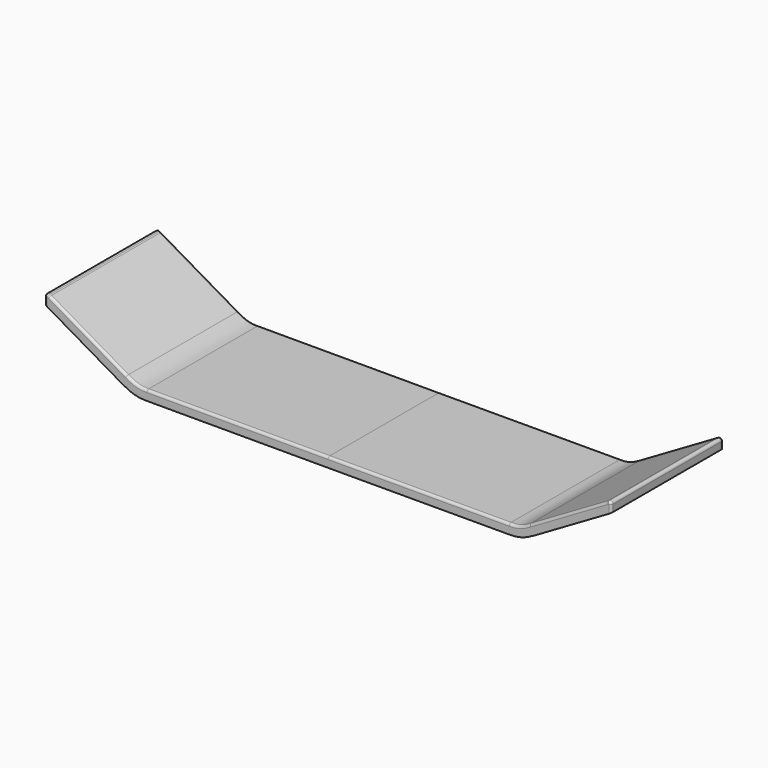
from build123d import *

# Parameters (mm, degrees)
F1_DEPTH = 146.05
F2_R     = 2.54


with BuildPart() as f1:
    # F0 (on Front) → F1 (new body)
    with BuildSketch(Plane.XZ):
        with BuildLine():
            Line((1.5943159571, 65.9026825806), (1.5943159571, 54.15516499))
            Line((1.5943159571, 54.15516499), (81.9025710225, 7.5405244716))
            add(Edge.make_bspline(
                [(81.9025710225, 7.5405244716), (92.2999233007, 1.5054497635), (98.6241698265, 0), (108.1725358963, 0)],
                knots=[0, 0, 0, 0, 27.3307622246, 27.3307622246, 27.3307622246, 27.3307622246], degree=3))
            Line((108.1725358963, 0), (138.4361670146, -1.768e-06))
            Line((138.4361670146, -1.768e-06), (163.8361670146, -3.2519e-06))
            Line((163.8361670146, -3.2519e-06), (297.1861670146, -1.10422e-05))
            Line((297.1861670146, -1.10422e-05), (297.1800001915, 10.1599889582))
            Line((297.1800001915, 10.1599889582), (108.1725311829, 10.16))
            add(Edge.make_bspline(
                [(87.0029644932, 16.3275368446), (88.188553852, 15.6393696939), (90.394248444, 14.4210715589), (93.2713691382, 13.0231304302), (95.7978416249, 11.994384017), (98.0869107324, 11.2602812726), (100.2922847586, 10.7469020057), (102.5915460742, 10.4019914085), (105.1499671195, 10.2020688941), (107.1124775165, 10.1600000624), (108.1725311829, 10.16)],
                knots=[7.877e-07, 7.877e-07, 7.877e-07, 7.877e-07, 0.125, 0.25, 0.375, 0.5, 0.625, 0.75, 0.875, 0.9999998147, 0.9999998147, 0.9999998147, 0.9999998147], degree=3))
            Line((87.0029644932, 16.3275368446), (6.6947068499, 62.9421788594))
            Line((6.6947068499, 62.9421788594), (1.5943159571, 65.9026825806))
        make_face()
    extrude(amount=F1_DEPTH)

    # F2
    f2_edges = [f1.edges().sort_by_distance(p)[0] for p in [
        (202.676266, 0, 10.159994),
        (97.116174, 0, 11.580578),
        (44.29864, 0, 41.11511),
        (1.594316, -73.025, 65.902683),
        (44.29864, -146.05, 41.11511),
        (97.116174, -146.05, 11.580578),
        (202.676266, -146.05, 10.159994),
        (1.594316, -146.05, 60.028924),
        (1.594316, 0, 60.028924),
    ]]
    fillet(f2_edges, radius=F2_R)

    # F3: F1 across face


with BuildPart() as f1_1:
    add(f1.part)
    add(f1.part.mirror(Plane(origin=(297.1830887239, -73.025, 5.0715521532), x_dir=(0, 1, 0), z_dir=(0.9999998158, 0, 0.0006069707))))


with BuildPart() as f4_1:
    # F4: copy of F1
    add(f1_1.part.moved(Location((0, 190.5, 0))))


with BuildPart() as f5_1:
    # F5: copy of F4_1
    add(f4_1.part.moved(Location((0, 190.5, 0))))


with BuildPart() as f6_1:
    # F6: copy of F5_1
    add(f5_1.part.moved(Location((0, 190.5, 0))))


solid = f1_1.part
